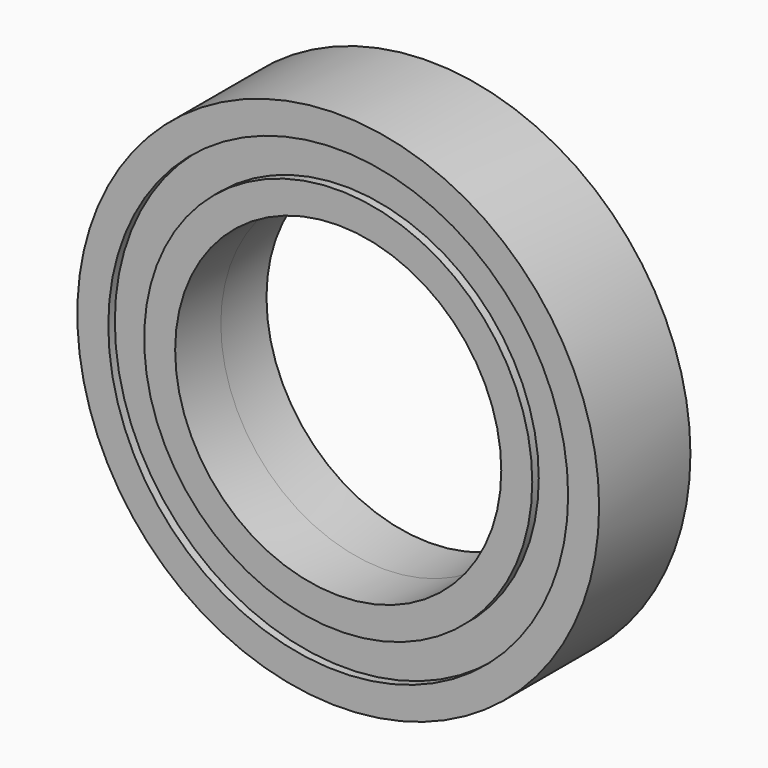
from build123d import *

# Parameters (mm, degrees)
F0_R          = 16
F0_R_2        = 10
F1_DEPTH      = 3.5
F1_DEPTH_BACK = 3.5
F2_R          = 14.1
F2_R_2        = 11.9
F3_DEPTH      = 0.5


# Not quite as in the source:
# - a pattern or mirror of a feature is missing from the dataset's text; its kind, count and spacing are read off the source's solid


with BuildPart() as f1:
    # F0 (on Front) → F1 (new body, two sides)
    with BuildSketch(Plane.XZ) as f1_sk:
        Circle(F0_R)
        Circle(F0_R_2, mode=Mode.SUBTRACT)
    extrude(amount=F1_DEPTH)
    extrude(f1_sk.sketch, amount=-F1_DEPTH_BACK)

    # F2 (on face) → F3 (cut)
    with BuildSketch(Plane.XZ.offset(3.5)):
        Circle(F2_R)
        Circle(F2_R_2, mode=Mode.SUBTRACT)
    f3 = extrude(amount=-F3_DEPTH, mode=Mode.SUBTRACT)

    # F3_copies: F3 across plane
    add(f3.mirror(Plane.ZX), mode=Mode.SUBTRACT)


solid = f1.part
